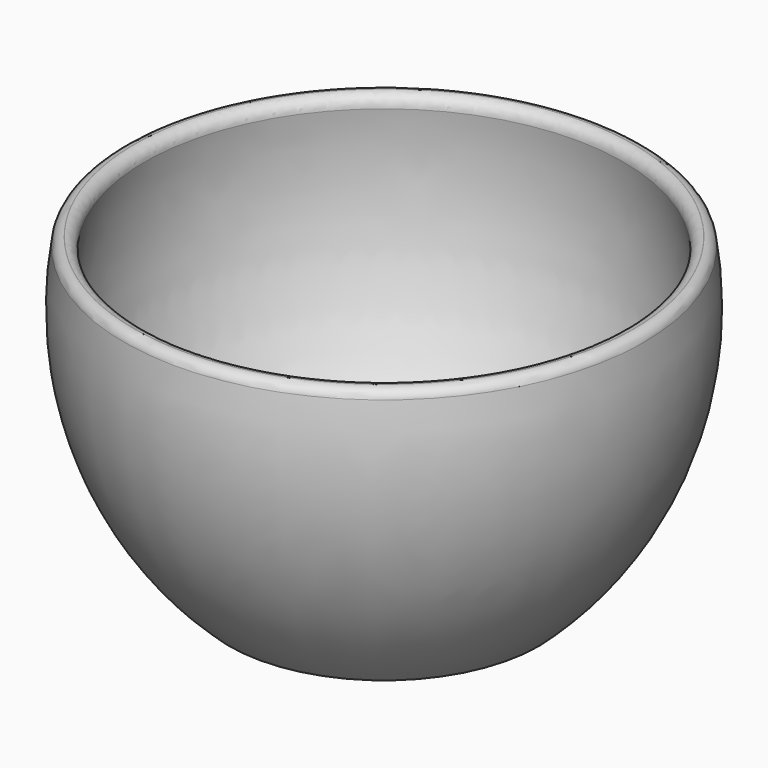
from build123d import *

# Parameters (mm, degrees)
F2_T     = -4
F4_ANGLE = 90
F6_R     = 2


# Not quite as in the source:
# - a fillet or chamfer that OpenCascade refuses, or shapes differently, is made with other operations: its cross-section is extruded or revolved along the edge and cut away or added


with BuildPart() as f1:
    # F0 (on Top) → F1 (revolve)
    with BuildSketch(Plane.XY):
        with BuildLine():
            Line((0, 60), (0, 0))
            Line((0, 0), (30, 0))
            ThreePointArc((30, 0), (47.7751027914, 27.4082990695), (50, 60))
            Line((50, 60), (0, 60))
        make_face()
    revolve(axis=Axis((0, 30, 0), (0, 1, 0)))

    # F2
    f2_openings = [f1.faces().sort_by_distance(p)[0] for p in [
        (0, 60, 0),
    ]]
    offset(amount=F2_T, openings=f2_openings)


with BuildPart() as f1_1:
    # F4: moved
    add(f1.part.rotate(Axis((-0.2157390118, 0, 0), (1, 0, 0)), F4_ANGLE))

    # F5: fillet of radius 2 on 2 edges, made by hand

    # F5_s1 → F5_t2 (revolve, cut)
    with BuildSketch(Plane.XZ):
        with BuildLine():
            ThreePointArc((50.2934782333, 58.3159438732), (49.61547632, 59.5221562829), (48.3170473003, 60.0004))
            Line((48.3170473003, 60.0004), (48.3170473003, 60.2005735625))
            ThreePointArc((48.3170473003, 60.2005735625), (49.1585236502, 60.2001735625), (50, 60.2001735625))
            Line((50, 60.2001735625), (50.19674198, 60.0369059404))
            ThreePointArc((50.19674198, 60.0369059404), (50.3492792076, 59.1932194953), (50.4911213266, 58.347671823))
            Line((50.4911213266, 58.347671823), (50.2934782333, 58.3159438732))
        make_face()
    revolve(axis=Axis((0, 0, 60), (0, 0, 1)), mode=Mode.SUBTRACT)

    # F5_s3 → F5_t4 (revolve, cut)
    with BuildSketch(Plane.XZ):
        with BuildLine():
            ThreePointArc((48.3190144803, 60.0004), (46.7959979699, 59.2973105964), (46.343205957, 57.6821036767))
            Line((46.343205957, 57.6821036767), (46.1456251047, 57.6503847263))
            ThreePointArc((46.1456251047, 57.6503847263), (45.948875499, 58.8071718158), (45.7335516417, 59.9631056529))
            Line((45.7335516417, 59.9631056529), (45.9302318191, 60.2001106819))
            ThreePointArc((45.9302318191, 60.2001106819), (47.1246231497, 60.2001106819), (48.3190144803, 60.2005106819))
            Line((48.3190144803, 60.2005106819), (48.3190144803, 60.0004))
        make_face()
    revolve(axis=Axis((-2.349e-07, -3e-10, 60), (0, 0, -1)), mode=Mode.SUBTRACT)

    # F6
    f6_edges = [f1_1.edges().sort_by_distance(p)[0] for p in [
        (-45.930232, 0, 60),
    ]]
    fillet(f6_edges, radius=F6_R)


solid = f1_1.part
